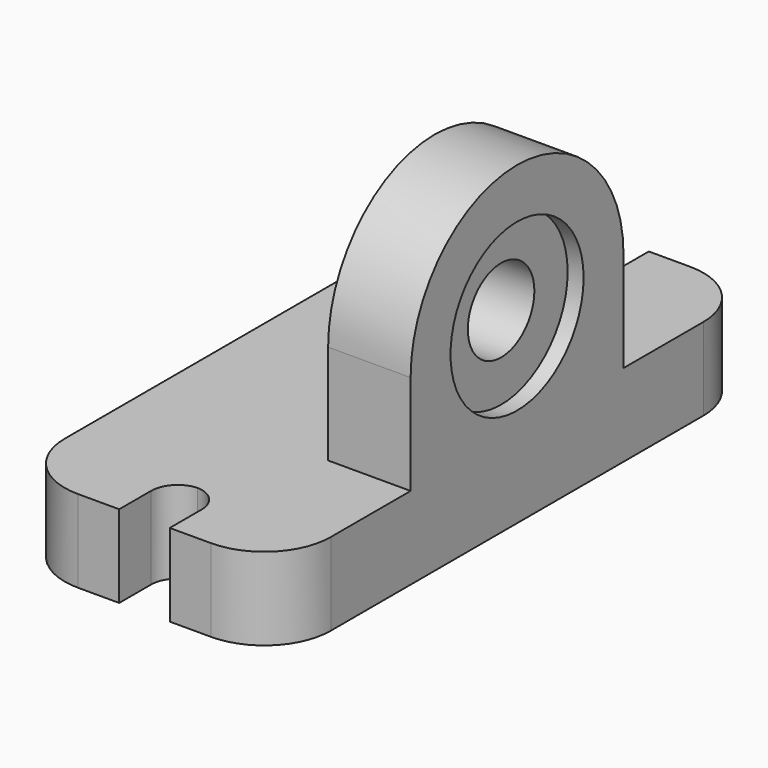
from build123d import *

# Parameters (mm, degrees)
F0_W        = 50.8
F0_H        = 114.3
F1_DEPTH    = 15.748
F2_W        = 9.652
F2_H        = 12.7
F3_DEPTH    = 25.4
F4_R        = 12.7
F5_T1_DEPTH = 15.748
F7_DEPTH    = 15.748
F8_R        = 15.875
F9_DEPTH    = 3.048
F10_R       = 7.9375
F11_DEPTH   = 25.4


# Not quite as in the source:
# - a fillet or chamfer that OpenCascade refuses, or shapes differently, is made with other operations: its cross-section is extruded or revolved along the edge and cut away or added


with BuildPart() as f1:
    # F0 (on Top) → F1 (new body)
    with BuildSketch(Plane.XY):
        with Locations((-2.3709591478, 9.3886919219)):
            Rectangle(F0_W, F0_H)
    extrude(amount=F1_DEPTH)

    # F2 (on face) → F3 (cut)
    with BuildSketch(Plane.XY.offset(15.748)):
        with Locations((-2.3709591478, -41.4113080781)):
            Rectangle(F2_W, F2_H)
        with Locations((-2.3709591478, 60.1886919219)):
            Rectangle(F2_W, F2_H)
    extrude(amount=-F3_DEPTH, mode=Mode.SUBTRACT)

    # F4
    f4_edges = [f1.edges().sort_by_distance(p)[0] for p in [
        (-27.770959, 66.538692, 7.874),
        (23.029041, 66.538692, 7.874),
        (-27.770959, -47.761308, 7.874),
        (23.029041, -47.761308, 7.874),
    ]]
    fillet(f4_edges, radius=F4_R)

    # F5: fillet of radius 5.08 on 4 edges, made by hand

    # F5_s2 → F5_t1 (join)
    with BuildSketch(Plane.XY):
        with BuildLine():
            ThreePointArc((-2.6249591478, 53.8386919219), (0.9671433006, 55.3265894735), (2.4550408522, 58.9186919219))
            Line((2.4550408522, 58.9186919219), (2.4550408522, 53.8386919219))
            Line((2.4550408522, 53.8386919219), (-2.6249591478, 53.8386919219))
        make_face()
        with BuildLine():
            ThreePointArc((-7.1969591478, 58.9186919219), (-5.7090615962, 55.3265894735), (-2.1169591478, 53.8386919219))
            Line((-2.1169591478, 53.8386919219), (-7.1969591478, 53.8386919219))
            Line((-7.1969591478, 53.8386919219), (-7.1969591478, 58.9186919219))
        make_face()
        with BuildLine():
            ThreePointArc((-2.6249591478, -35.0613080781), (0.9671433006, -36.5492056297), (2.4550408522, -40.1413080781))
            Line((2.4550408522, -40.1413080781), (2.4550408522, -35.0613080781))
            Line((2.4550408522, -35.0613080781), (-2.6249591478, -35.0613080781))
        make_face()
        with BuildLine():
            ThreePointArc((-7.1969591478, -40.1413080781), (-5.7090615962, -36.5492056297), (-2.1169591478, -35.0613080781))
            Line((-2.1169591478, -35.0613080781), (-7.1969591478, -35.0613080781))
            Line((-7.1969591478, -35.0613080781), (-7.1969591478, -40.1413080781))
        make_face()
    extrude(amount=F5_T1_DEPTH)

    # F6 (on face) → F7 (join)
    with BuildSketch(Plane.YZ.offset(23.0290408522)):
        with BuildLine():
            Line((34.7886919219, 15.748), (34.7886919219, 34.798))
            ThreePointArc((34.7886919219, 34.798), (9.3886919219, 60.198), (-16.0113080781, 34.798))
            Line((-16.0113080781, 34.798), (-16.0113080781, 15.748))
            Line((-16.0113080781, 15.748), (34.7886919219, 15.748))
        make_face()
    extrude(amount=-F7_DEPTH)

    # F8 (on face) → F9 (cut)
    with BuildSketch(Plane.YZ.offset(23.0290408522)):
        with Locations((9.3886919219, 34.798)):
            Circle(F8_R)
    extrude(amount=-F9_DEPTH, mode=Mode.SUBTRACT)

    # F10 (on face) → F11 (cut)
    with BuildSketch(Plane.YZ.offset(19.9810408522)):
        with Locations((9.3886919219, 34.798)):
            Circle(F10_R)
    extrude(amount=-F11_DEPTH, mode=Mode.SUBTRACT)


solid = f1.part
